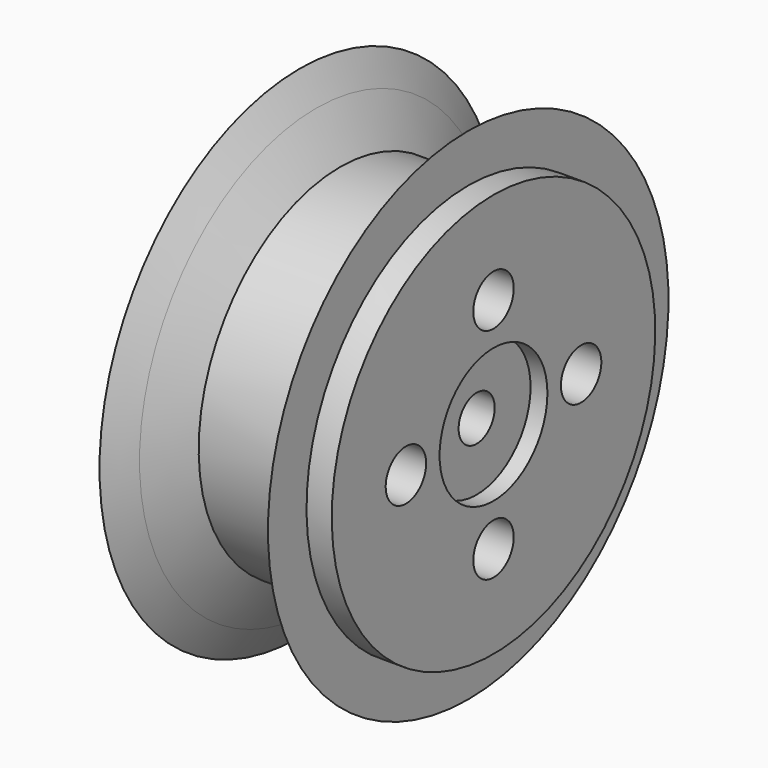
from build123d import *

# Parameters (mm, degrees)
F0_W     = 4.7625
F0_H     = 38.1
F2_R     = 4.25
F3_DEPTH = 36.5135
F2_R_2   = 12.7
F4_DEPTH = 3.175
F5_R     = 12.7
F5_R_2   = 4.25
F6_DEPTH = 3.175
F5_R_3   = 4.7625
F7_DEPTH = 36.5135


with BuildPart() as f1:
    # F0 (on Front) → F1 (revolve)
    with BuildSketch(Plane.XZ):
        with BuildLine():
            Line((-12.8016, 41.5925), (-15.875, 41.5925))
            Line((-15.875, 41.5925), (-15.875, 0))
            Line((-15.875, 0), (-4.7625, 0))
            ThreePointArc((-4.7625, 0), (0, 4.7625), (4.7625, 0))
            Line((4.7625, 0), (15.875, 0))
            Line((15.875, 0), (15.875, 38.1))
            Line((15.875, 38.1), (15.875, 41.5925))
            Line((15.875, 41.5925), (12.8016, 41.5925))
            Line((12.8016, 41.5925), (8.255, 33.3375))
            Line((8.255, 33.3375), (-8.255, 33.3375))
            Line((-8.255, 33.3375), (-12.8016, 41.5925))
        make_face()
        with Locations((18.25625, 19.05)):
            Rectangle(F0_W, F0_H)
        with BuildLine():
            ThreePointArc((4.7625, 0), (0, 4.7625), (-4.7625, 0))
            Line((-4.7625, 0), (4.7625, 0))
        make_face()
        Polygon((-15.875, 47.1726955307), (-15.875, 41.5925), (-12.8016, 41.5925), align=None)
        Polygon((15.875, 47.1726955307), (12.8016, 41.5925), (15.875, 41.5925), align=None)
    revolve(axis=Axis((2.38125, 0, 0), (1, 0, 0)))

    # F2 (on face) → F3 (cut, through all)
    with BuildSketch(Plane.YZ.offset(20.6375)):
        Circle(F2_R)
    extrude(amount=-F3_DEPTH, mode=Mode.SUBTRACT)

    # F2 (on face) → F4 (cut)
    with BuildSketch(Plane.YZ.offset(20.6375)):
        Circle(F2_R_2)
        Circle(F2_R, mode=Mode.SUBTRACT)
    extrude(amount=-F4_DEPTH, mode=Mode.SUBTRACT)

    # F5 (on face) → F6 (cut)
    with BuildSketch(Plane(origin=(-15.875, 0, 0), x_dir=(0, -1, 0), z_dir=(-1, 0, 0))):
        Circle(F5_R)
        Circle(F5_R_2, mode=Mode.SUBTRACT)
        Circle(F5_R_2)
    extrude(amount=-F6_DEPTH, mode=Mode.SUBTRACT)

    # F5 (on face) → F7 (cut, through all)
    with BuildSketch(Plane(origin=(-15.875, 0, 0), x_dir=(0, -1, 0), z_dir=(-1, 0, 0))):
        with Locations((0, 20.6375)):
            Circle(F5_R_3)
        with Locations((20.6375, 0)):
            Circle(F5_R_3)
        with Locations((0, -20.6375)):
            Circle(F5_R_3)
        with Locations((-20.6375, 0)):
            Circle(F5_R_3)
    extrude(amount=-F7_DEPTH, mode=Mode.SUBTRACT)


solid = f1.part
